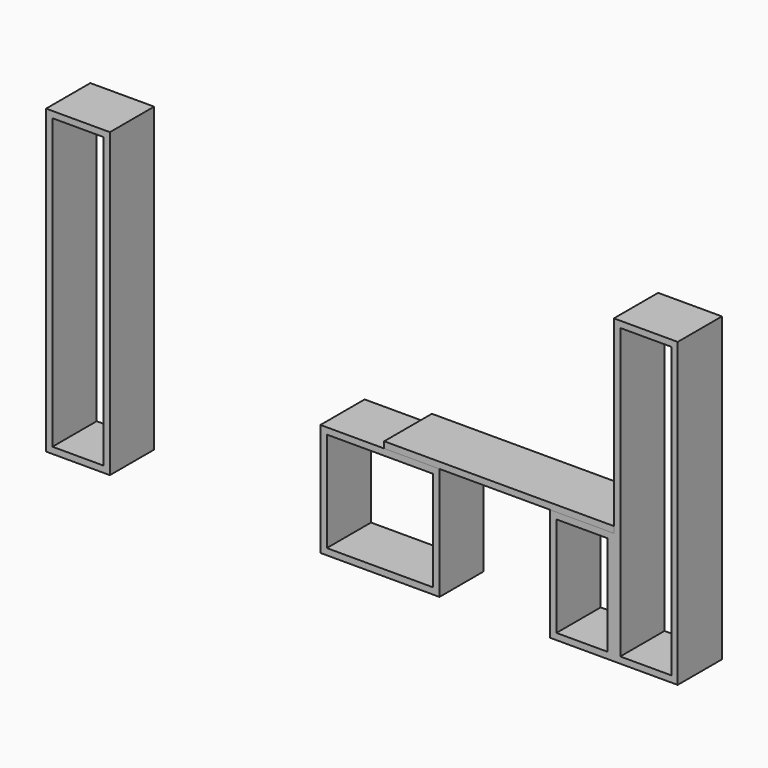
from build123d import *

# Parameters (mm, degrees)
F0_W     = 381
F0_H     = 1803.4
F0_W_2   = 304.8
F0_H_2   = 1727.2
F1_DEPTH = 330.2
F0_W_3   = 635
F0_H_3   = 596.9
F0_H_4   = 673.1
F3_DEPTH = 355.6


# Not quite as in the source:
# - a feature names something its author has since deleted; it is built from what else it names


with BuildPart() as f1:
    # F0 (on Front) → F1 (new body)
    with BuildSketch(Plane.XZ):
        with Locations((-3581.4, 901.7)):
            Rectangle(F0_W, F0_H)
        with Locations((-3581.4, 901.7)):
            Rectangle(F0_W_2, F0_H_2, mode=Mode.SUBTRACT)
    extrude(amount=F1_DEPTH)


with BuildPart() as f1b:
    # F0 (on Front) → F1, piece 2 (new body)
    with BuildSketch(Plane.XZ):
        Polygon((-2133.6, 673.1), (-2133.6, 0), (-1752.6, 0), (-1422.4, 0), (-1422.4, 673.1), (-1752.6, 673.1), (-1790.7, 673.1), (-2095.5, 673.1), align=None)
        with Locations((-1778, 336.55)):
            Rectangle(F0_W_3, F0_H_3, mode=Mode.SUBTRACT)
    extrude(amount=F1_DEPTH)


with BuildPart() as f1c:
    # F0 (on Front) → F1, piece 3 (new body)
    with BuildSketch(Plane.XZ):
        with Locations((-571.5, 336.55)):
            Rectangle(F0_W, F0_H_4)
        with Locations((-571.5, 336.55)):
            Rectangle(F0_W_2, F0_H_3, mode=Mode.SUBTRACT)
        Polygon((-38.1, 0), (0, 0), (0, 1803.4), (-38.1, 1803.4), (-342.9, 1803.4), (-381, 1803.4), (-381, 673.1), (-381, 0), (-342.9, 0), align=None)
        with Locations((-190.5, 901.7)):
            Rectangle(F0_W_2, F0_H_2, mode=Mode.SUBTRACT)
    extrude(amount=F1_DEPTH)


with BuildPart() as f3:
    # F2 (on face) → F3 (new body)
    with BuildSketch(Plane.XZ.offset(330.2)):
        Polygon((-1752.6, 711.2), (-1752.6, 673.1), (-1422.4, 673.1), (-381, 673.1), (-381, 711.2), align=None)
    extrude(amount=-F3_DEPTH)


solid = Compound([f1.part, f1b.part, f1c.part, f3.part])
